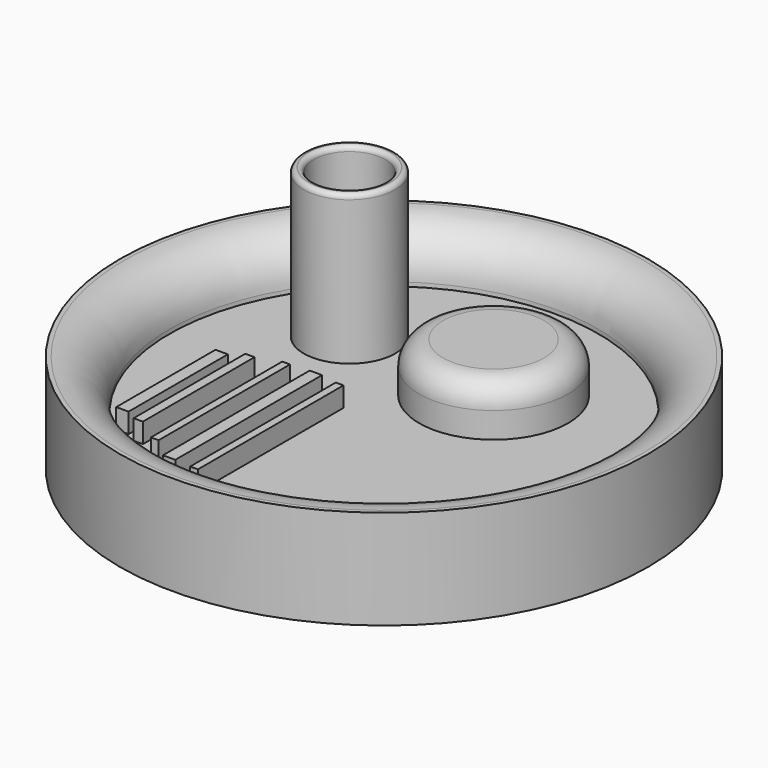
from build123d import *

# Parameters (mm, degrees)
F0_R      = 67.5268946045
F1_DEPTH  = 25.4
F2_T      = -12.7
F3_R      = 11.650994652
F4_R      = 19.05
F5_DEPTH  = 12.7
F6_R      = 6.1321024484
F8_R      = 11.7086164589
F9_DEPTH  = 38.1
F10_T     = 2.54
F11_R     = 1.2264204897
F7_W      = 3.1531006098
F7_H      = 31.7281037569
F7_W_2    = 2.3648291826
F7_H_2    = 35.6694851071
F7_W_3    = 1.9706897438
F7_H_3    = 41.9756902847
F7_W_4    = 3.1531024724
F7_H_4    = 46.902414877
F7_W_5    = 1.9706902094
F7_H_5    = 46.5082784649
F12_DEPTH = 5.08


# Not quite as in the source:
# - a shell that OpenCascade refuses in one call is made with other operations: the cavity is built on its own and cut out


with BuildPart() as f1:
    # F0 (on Top) → F1 (new body)
    with BuildSketch(Plane.XY):
        Circle(F0_R)
    extrude(amount=F1_DEPTH)

    # F2
    f2_openings = [f1.faces().sort_by_distance(p)[0] for p in [
        (0, 0, 25.4),
    ]]
    offset(amount=F2_T, openings=f2_openings)

    # F3
    f3_edges = [f1.edges().sort_by_distance(p)[0] for p in [
        (-54.826895, 0, 25.4),
    ]]
    fillet(f3_edges, radius=F3_R)

    # F4 (on face) → F5 (join)
    with BuildSketch(Plane.XY.offset(12.7)):
        with Locations((12.4153438956, 19.5098277181)):
            Circle(F4_R)
    extrude(amount=F5_DEPTH)

    # F6
    f6_edges = [f1.edges().sort_by_distance(p)[0] for p in [
        (-6.634656, 19.509828, 25.4),
    ]]
    fillet(f6_edges, radius=F6_R)

    # F8 (on face) → F9 (join)
    with BuildSketch(Plane.XY.offset(12.7)):
        with Locations((-26.0131042451, 21.4805174619)):
            Circle(F8_R)
    extrude(amount=F9_DEPTH)

    # F10: shell of thickness 2.54, made by hand


with BuildPart() as f10_core1:
    # F10_t2: copy of F1
    add(f1.part)

    # the walls: a layer under each face that stays
    f10_faces = [f10_core1.faces().sort_by_distance(p)[0] for p in [
        (-6.6346561044, 19.5098277181, 15.9839487758),
        (-4.8386048802, 19.5098277181, 23.6039487758),
        (0, 0, 12.7),
        (12.4153438956, 19.5098277181, 25.4),
        (-54.8268946045, 0, 13.224502674),
        (-37.721720704, 21.4805174619, 31.75),
        (-58.2393919305, 0, 21.987502674),
        (59.0860327789, -32.512949254, 25.4),
        (-67.5268946045, 0, 12.7),
        (0, 0, 0),
    ]]
    thicken(f10_faces, amount=-F10_T, mode=Mode.SUBTRACT)

    # F10_s3 → F10_t4 (revolve, cut)
    with BuildSketch(Plane.XZ.offset(-19.5098277181)):
        Polygon((31.4907438956, 12.7254), (28.9253438956, 12.7), (28.9253438956, 10.16), (31.4653438956, 10.16), align=None)
    revolve(axis=Axis((12.4153438956, 19.5098277181, 12.7), (0, 0, 1)), mode=Mode.SUBTRACT)

    # F10_s5 → F10_t6 (revolve, cut)
    with BuildSketch(Plane.XZ):
        Polygon((54.8014946045, 12.7254), (54.8268946045, 10.16), (57.3668946045, 10.16), (57.3668946045, 12.7), align=None)
    revolve(axis=Axis((0, 0, 12.7), (0, 0, -1)), mode=Mode.SUBTRACT)

    # F10_s7 → F10_t8 (revolve, cut)
    with BuildSketch(Plane.XZ.offset(-21.4805174619)):
        Polygon((-14.2790877862, 12.7254), (-14.3044877862, 10.16), (-16.8444877862, 10.16), (-16.8444877862, 12.7), align=None)
    revolve(axis=Axis((-26.0131042451, 21.4805174619, 12.7), (0, 0, 1)), mode=Mode.SUBTRACT)


with BuildPart() as f1_1:
    add(f1.part)

    # what is left inside the walls is the cavity
    f10_cavity = [f10_core1.part.solids().sort_by_distance(p)[0] for p in [
        (0, -21.662298, 2.5654),
    ]]
    add(f10_cavity, mode=Mode.SUBTRACT)

    # F11
    f11_edges = [f1_1.edges().sort_by_distance(p)[0] for p in [
        (-37.721721, 21.480517, 50.8),
        (-35.181721, 21.480517, 50.8),
    ]]
    fillet(f11_edges, radius=F11_R)

    # F7 (on face) → F12 (join)
    with BuildSketch(Plane.XY.offset(12.7)):
        with Locations((-35.6694832444, -23.1556035578)):
            Rectangle(F7_W, F7_H)
        with Locations((-30.3486213088, -22.7614669129)):
            Rectangle(F7_W_2, F7_H_2)
        with Locations((-22.6629320532, -23.9438795252)):
            Rectangle(F7_W_3, F7_H_3)
        with Locations((-15.3713794425, -26.0131040122)):
            Rectangle(F7_W_4, F7_H_4)
        with Locations((-8.671034826, -26.6043116571)):
            Rectangle(F7_W_5, F7_H_5)
    extrude(amount=F12_DEPTH)


solid = f1_1.part
